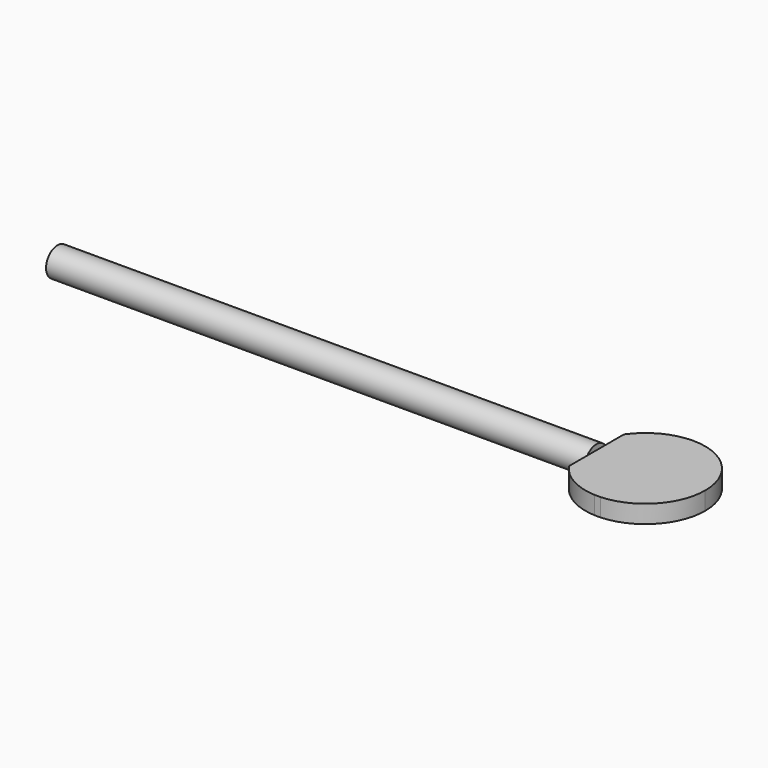
from build123d import *

# Parameters (mm, degrees)
F0_R     = 3.048
F1_DEPTH = 114.3
F3_DEPTH = 25.4
F5_DEPTH = 25.4


with BuildPart() as f1:
    # F0 (on Right) → F1 (new body)
    with BuildSketch(Plane.YZ):
        Circle(F0_R)
    extrude(amount=F1_DEPTH)

    # F2 (on face) → F3 (join)
    with BuildSketch(Plane.YZ.offset(114.3)):
        with BuildLine():
            Line((-12.6839943098, -1.8982821818), (-2.3847072689, -1.8982821818))
            ThreePointArc((-2.3847072689, -1.8982821818), (-3.0479878513, 0.0086057166), (-2.3739500803, 1.9117178182))
            Line((-2.3739500803, 1.9117178182), (-12.6839943098, 1.9117178182))
            Line((-12.6839943098, 1.9117178182), (-12.6839943098, -1.8982821818))
        make_face()
        with BuildLine():
            Line((-2.3847072689, -1.8982821818), (2.3847072689, -1.8982821818))
            ThreePointArc((2.3847072689, -1.8982821818), (2.877402627, -1.0054144032), (3.048, 0))
            ThreePointArc((3.048, 0), (2.8745524734, 1.0135344482), (2.3739500803, 1.9117178182))
            Line((2.3739500803, 1.9117178182), (-2.3739500803, 1.9117178182))
            ThreePointArc((-2.3739500803, 1.9117178182), (-3.0479878513, 0.0086057166), (-2.3847072689, -1.8982821818))
        make_face()
        with BuildLine():
            Line((2.3847072689, -1.8982821818), (12.7160056902, -1.8982821818))
            Line((12.7160056902, -1.8982821818), (12.7160056902, 1.9117178182))
            Line((12.7160056902, 1.9117178182), (2.3739500803, 1.9117178182))
            ThreePointArc((2.3739500803, 1.9117178182), (2.8745524734, 1.0135344482), (3.048, 0))
            ThreePointArc((3.048, 0), (2.877402627, -1.0054144032), (2.3847072689, -1.8982821818))
        make_face()
    extrude(amount=F3_DEPTH)

    # F4 (on face) → F5 (cut)
    with BuildSketch(Plane.XY.offset(1.9117178182)):
        with BuildLine():
            ThreePointArc((114.3, 7.3106571527), (128.51905795, 12.1073757501), (137.3848106384, 0))
            ThreePointArc((137.3848106384, 0), (133.8876655087, -8.751997614), (125.3222181603, -12.6839943098))
            Line((125.3222181603, -12.6839943098), (139.7, -12.6839943098))
            Line((139.7, -12.6839943098), (139.7, 12.7160056902))
            Line((139.7, 12.7160056902), (114.3, 12.7160056902))
            Line((114.3, 12.7160056902), (114.3, 7.3106571527))
        make_face()
        with BuildLine():
            ThreePointArc((124.0474031165, -12.6839943098), (118.5537005151, -11.1220271828), (114.3, -7.3106571527))
            Line((114.3, -7.3106571527), (114.3, -12.6839943098))
            Line((114.3, -12.6839943098), (124.0474031165, -12.6839943098))
        make_face()
    extrude(amount=-F5_DEPTH, mode=Mode.SUBTRACT)


solid = f1.part
